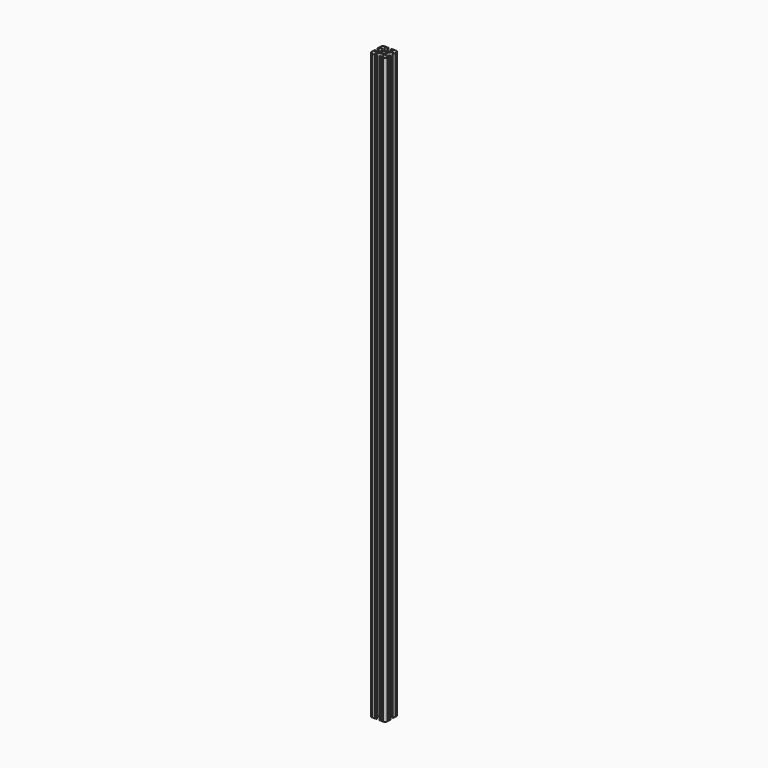
from build123d import *

# Parameters (mm, degrees)
F0_R     = 3.3625011168
F1_DEPTH = 939.8


# Not quite as in the source:
# - ends of sketch curves that miss each other by under 0.0002 mm in the source are joined


with BuildPart() as f1:
    # F0 (on Top) → F1 (new body)
    with BuildSketch(Plane.XY):
        with BuildLine():
            ThreePointArc((-8.5485764575, 18.7552378401), (-9.7846294165, 17.9293336576), (-11.2426532939, 17.6393146764))
            Line((-11.2426532939, 17.6393146764), (-14.1573467061, 17.6393146764))
            ThreePointArc((-14.1573467061, 17.6393146764), (-15.6153705835, 17.9293336576), (-16.8514235425, 18.7552378401))
            Line((-16.8514235425, 18.7552378401), (-18.696905198, 20.6007194956))
            ThreePointArc((-18.696905198, 20.6007194956), (-19.1098572893, 22.6767698525), (-17.3498667798, 23.8527579138))
            Line((-17.3498667798, 23.8527579138), (-15.6153705835, 23.8527579138))
            Line((-15.6153705835, 23.8527579138), (-15.5830195394, 23.8527579138))
            ThreePointArc((-15.5830195394, 23.8527579138), (-14.8254049311, 24.6263789569), (-15.5830195394, 25.4))
            Line((-15.5830195394, 25.4), (-15.6153705835, 25.4))
            Line((-15.6153705835, 25.4), (-16.2533409894, 25.4))
            ThreePointArc((-16.2533409894, 25.4), (-16.8016038846, 24.8587722652), (-17.3498667798, 25.4))
            Line((-17.3498667798, 25.4), (-20.4874817282, 25.4))
            ThreePointArc((-20.4874817282, 25.4), (-21.0387408641, 24.8487408595), (-21.5900000046, 25.4))
            ThreePointArc((-21.5900000046, 25.4), (-24.2840768363, 24.2840768363), (-25.4, 21.59))
            Line((-25.4, 21.59), (-25.4, 20.5047242343))
            Line((-25.4, 20.5047242343), (-25.4, 17.3498667798))
            ThreePointArc((-25.4, 17.3498667798), (-24.8441605755, 16.8026749055), (-25.4, 16.2554830313))
            Line((-25.4, 16.2554830313), (-25.4, 15.6153705835))
            ThreePointArc((-25.4, 15.6153705835), (-24.6263789569, 14.8595541131), (-23.8527579138, 15.6153705835))
            Line((-23.8527579138, 15.6153705835), (-23.8527579138, 17.3498667798))
            ThreePointArc((-23.8527579138, 17.3498667798), (-22.6767698525, 19.1098572893), (-20.6007194956, 18.696905198))
            Line((-20.6007194956, 18.696905198), (-18.7552378401, 16.8514235425))
            ThreePointArc((-18.7552378401, 16.8514235425), (-17.9293336576, 15.6153705835), (-17.6393146764, 14.1573467061))
            Line((-17.6393146764, 14.1573467061), (-17.6393146764, 11.2426532939))
            ThreePointArc((-17.6393146764, 11.2426532939), (-17.9293336576, 9.7846294165), (-18.7552378401, 8.5485764575))
            Line((-18.7552378401, 8.5485764575), (-20.6007194956, 6.703094802))
            ThreePointArc((-20.6007194956, 6.703094802), (-22.6767698525, 6.2901427107), (-23.8527579138, 8.0501332202))
            Line((-23.8527579138, 8.0501332202), (-23.8527579138, 9.7846294165))
            ThreePointArc((-23.8527579138, 9.7846294165), (-24.6263789569, 10.5582546272), (-25.4000041675, 9.7846294165))
            Line((-25.4000041675, 9.7846294165), (-25.4, 9.1492393985))
            ThreePointArc((-25.4, 9.1492393985), (-24.8993742936, 8.5996863094), (-25.4, 8.0501332202))
            Line((-25.4, 8.0501332202), (-25.4, 4.904538393))
            ThreePointArc((-25.4, 4.904538393), (-24.8462160257, 4.3572691965), (-25.4, 3.81))
            ThreePointArc((-25.4, 3.81), (-24.2840768363, 1.1159231637), (-21.59, 0))
            ThreePointArc((-21.59, 0), (-21.0408167821, 0.5548848314), (-20.4916335642, 0))
            Line((-20.4916335642, 0), (-16.7081691325, 0))
            ThreePointArc((-16.7081691325, 0), (-16.161769858, 0.5401345174), (-15.6153705835, 0))
            ThreePointArc((-15.6153705835, 0), (-14.8541835334, 0.7747), (-15.6153705835, 1.5494))
            Line((-15.6153705835, 1.5494), (-17.347708866, 1.5494))
            ThreePointArc((-17.347708866, 1.5494), (-19.1076993754, 2.7253880613), (-18.6947472842, 4.8014384182))
            Line((-18.6947472842, 4.8014384182), (-16.8514235425, 6.6447621599))
            ThreePointArc((-16.8514235425, 6.6447621599), (-15.6153705835, 7.4706663424), (-14.1573467061, 7.7606853236))
            Line((-14.1573467061, 7.7606853236), (-11.2426532939, 7.7606853236))
            ThreePointArc((-11.2426532939, 7.7606853236), (-9.7846294165, 7.4706663424), (-8.5485764575, 6.6447621599))
            Line((-8.5485764575, 6.6447621599), (-6.7052527158, 4.8014384182))
            ThreePointArc((-6.7052527158, 4.8014384182), (-6.2923006246, 2.7253880613), (-8.052291134, 1.5494))
            Line((-8.052291134, 1.5494), (-9.7846294165, 1.5494))
            ThreePointArc((-9.7846294165, 1.5494), (-10.4018355229, 0.7747), (-9.7846294165, 0))
            Line((-9.7846294165, 0), (-9.1528678313, 0))
            ThreePointArc((-9.1528678313, 0), (-8.6025794826, 0.5452621138), (-8.052291134, 0))
            Line((-8.052291134, 0), (-4.8988661729, 0))
            ThreePointArc((-4.8988661729, 0), (-4.3544330864, 0.5444330864), (-3.81, 0))
            ThreePointArc((-3.81, 0), (-1.1159231637, 1.1159231637), (0, 3.81))
            ThreePointArc((0, 3.81), (-0.5393803924, 4.3561), (0, 4.9022))
            Line((0, 4.9022), (0, 8.052291134))
            ThreePointArc((0, 8.052291134), (-0.5435172497, 8.6016602673), (0, 9.1510294005))
            Line((0, 9.1510294005), (0, 9.7846294165))
            ThreePointArc((0, 9.7846294165), (-0.7747, 10.5046907664), (-1.5494, 9.7846294165))
            Line((-1.5494, 9.7846294165), (-1.5494, 8.052291134))
            ThreePointArc((-1.5494, 8.052291134), (-2.7253880613, 6.2923006246), (-4.8014384182, 6.7052527158))
            Line((-4.8014384182, 6.7052527158), (-6.6447621599, 8.5485764575))
            ThreePointArc((-6.6447621599, 8.5485764575), (-7.4706663424, 9.7846294165), (-7.7606853236, 11.2426532939))
            Line((-7.7606853236, 11.2426532939), (-7.7606853236, 14.1573467061))
            ThreePointArc((-7.7606853236, 14.1573467061), (-7.4706663424, 15.6153705835), (-6.6447621599, 16.8514235425))
            Line((-6.6447621599, 16.8514235425), (-4.8014384182, 18.6947472842))
            ThreePointArc((-4.8014384182, 18.6947472842), (-2.7253880613, 19.1076993754), (-1.5494, 17.347708866))
            Line((-1.5494, 17.347708866), (-1.5494, 15.6153705835))
            ThreePointArc((-1.5494, 15.6153705835), (-0.7747, 14.8794054827), (0, 15.6153705835))
            Line((0, 15.6153705835), (0, 16.255508866))
            ThreePointArc((0, 16.255508866), (-0.5461, 16.801608866), (0, 17.347708866))
            Line((0, 17.347708866), (0, 20.4951651394))
            ThreePointArc((0, 20.4951651394), (-0.5510556267, 21.0425825697), (0, 21.59))
            ThreePointArc((0, 21.59), (-1.1159231637, 24.2840768363), (-3.81, 25.4))
            ThreePointArc((-3.81, 25.4), (-4.3653028659, 24.9036192847), (-4.9206057318, 25.4))
            Line((-4.9206057318, 25.4), (-8.0501332202, 25.4))
            ThreePointArc((-8.0501332202, 25.4), (-8.5963647474, 24.8594330871), (-9.1425962746, 25.4))
            Line((-9.1425962746, 25.4), (-9.7846294165, 25.4))
            Line((-9.7846294165, 25.4), (-9.856202747, 25.4))
            ThreePointArc((-9.856202747, 25.4), (-10.594864404, 24.6263789569), (-9.856202747, 23.8527579138))
            Line((-9.856202747, 23.8527579138), (-9.7846294165, 23.8527579138))
            Line((-9.7846294165, 23.8527579138), (-8.0501332202, 23.8527579138))
            ThreePointArc((-8.0501332202, 23.8527579138), (-6.2901427107, 22.6767698525), (-6.703094802, 20.6007194956))
            Line((-6.703094802, 20.6007194956), (-8.5485764575, 18.7552378401))
        make_face()
        with Locations((-12.7, 12.7)):
            Circle(F0_R, mode=Mode.SUBTRACT)
        with BuildLine():
            ThreePointArc((-9.856202747, 23.8527579138), (-9.8204160818, 23.8519306347), (-9.7846294165, 23.8527579138))
            Line((-9.7846294165, 23.8527579138), (-9.856202747, 23.8527579138))
        make_face()
        with BuildLine():
            Line((-15.5830195394, 23.8527579138), (-15.6153705835, 23.8527579138))
            ThreePointArc((-15.6153705835, 23.8527579138), (-15.5991950614, 23.8525888265), (-15.5830195394, 23.8527579138))
        make_face()
        with BuildLine():
            ThreePointArc((-9.7846294165, 25.4), (-9.8204160818, 25.4008272791), (-9.856202747, 25.4))
            Line((-9.856202747, 25.4), (-9.7846294165, 25.4))
        make_face()
        with BuildLine():
            Line((-15.6153705835, 25.4), (-15.5830195394, 25.4))
            ThreePointArc((-15.5830195394, 25.4), (-15.5991950614, 25.4001690873), (-15.6153705835, 25.4))
        make_face()
    extrude(amount=F1_DEPTH)


solid = f1.part
